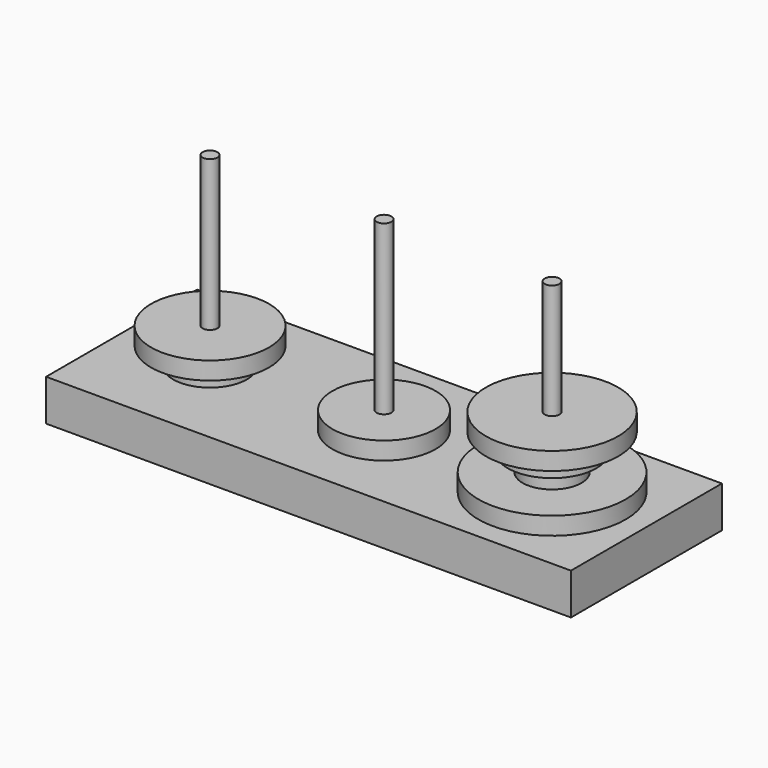
from build123d import *

# Parameters (mm, degrees)
F0_W      = 178
F0_H      = 14
F1_DEPTH  = 64
F3_R      = 2.5
F4_DEPTH  = 63
F6_E10_W  = 22.5
F6_E10_H  = 6
F9_E11_W  = 10
F9_E11_H  = 6
F9_E12_W  = 15
F9_E12_H  = 6
F13_E13_W = 7.5
F13_E13_H = 6
F16_E14_W = 17.5
F16_E14_H = 6
F19_E15_W = 12.5
F19_E15_H = 6
F22_E16_W = 20
F22_E16_H = 6


with BuildPart() as f1:
    # F0 (on Front) → F1 (new body)
    with BuildSketch(Plane.XZ):
        with Locations((133.2533232272, 56.5637208223)):
            Rectangle(F0_W, F0_H)
    extrude(amount=-F1_DEPTH)

    # F3 (on face) → F4 (join)
    with BuildSketch(Plane.XY.offset(63.5637208223)):
        with Locations((74.2533232272, 32)):
            Circle(F3_R)
        with Locations((133.2533232272, 32)):
            Circle(F3_R)
        with Locations((190.2533232272, 32)):
            Circle(F3_R)
    extrude(amount=F4_DEPTH)

    # F6_E10 (on explicit) → F7 (revolve)
    with BuildSketch(Plane(origin=(192.7533232272, 32, 63.5637208223), x_dir=(1, 0, 0), z_dir=(0, -1, 0))):
        with Locations((11.25, 3)):
            Rectangle(F6_E10_W, F6_E10_H)
    revolve(axis=Axis((190.2533232272, 32, 63.5637208223), (0, 0, -1)))

    # F9_E11 (on explicit) → F10 (revolve)
    with BuildSketch(Plane(origin=(71.7533232272, 32, 63.5637208223), x_dir=(-1, 0, 0), z_dir=(0, 1, 0))):
        with Locations((5, 3)):
            Rectangle(F9_E11_W, F9_E11_H)
    revolve(axis=Axis((74.2533232272, 32, 63.5637208223), (0, 0, -1)))

    # F13_E13 (on explicit) → F14 (revolve)
    with BuildSketch(Plane(origin=(187.9158168097, 32.886602362, 69.5637208223), x_dir=(-0.8739405908, 0.4860327599, 0), z_dir=(0.4860327599, 0.8739405908, 0))):
        with Locations((3.75, 3)):
            Rectangle(F13_E13_W, F13_E13_H)
    revolve(axis=Axis((190.2533232272, 32, 63.5637208223), (0, 0, -1)))

    # F16_E14 (on explicit) → F17 (revolve)
    with BuildSketch(Plane(origin=(76.7530926524, 31.9660467851, 69.5637208223), x_dir=(1, 0, 0), z_dir=(0, -1, 0))):
        with Locations((8.75, 3)):
            Rectangle(F16_E14_W, F16_E14_H)
    revolve(axis=Axis((74.2533232272, 32, 63.5637208223), (0, 0, -1)))

    # F19_E15 (on explicit) → F20 (revolve)
    with BuildSketch(Plane(origin=(192.7423164525, 32.2343346416, 75.5637208223), x_dir=(1, 0, 0), z_dir=(0, -1, 0))):
        with Locations((6.25, 3)):
            Rectangle(F19_E15_W, F19_E15_H)
    revolve(axis=Axis((190.2533232272, 32, 63.5637208223), (0, 0, -1)))

    # F22_E16 (on explicit) → F23 (revolve)
    with BuildSketch(Plane(origin=(187.8248049644, 32.5935478477, 81.5637208223), x_dir=(-1, 0, 0), z_dir=(0, 1, 0))):
        with Locations((10, 3)):
            Rectangle(F22_E16_W, F22_E16_H)
    revolve(axis=Axis((190.2533232272, 32, 63.5637208223), (0, 0, -1)))


with BuildPart() as f11:
    # F9_E12 (on explicit) → F11 (revolve)
    with BuildSketch(Plane(origin=(130.7533232272, 32, 63.5637208223), x_dir=(-1, 0, 0), z_dir=(0, 1, 0))):
        with Locations((7.5, 3)):
            Rectangle(F9_E12_W, F9_E12_H)
    revolve(axis=Axis((133.2533232272, 32, 63.5637208223), (0, 0, -1)))


solid = Compound([f1.part, f11.part])
